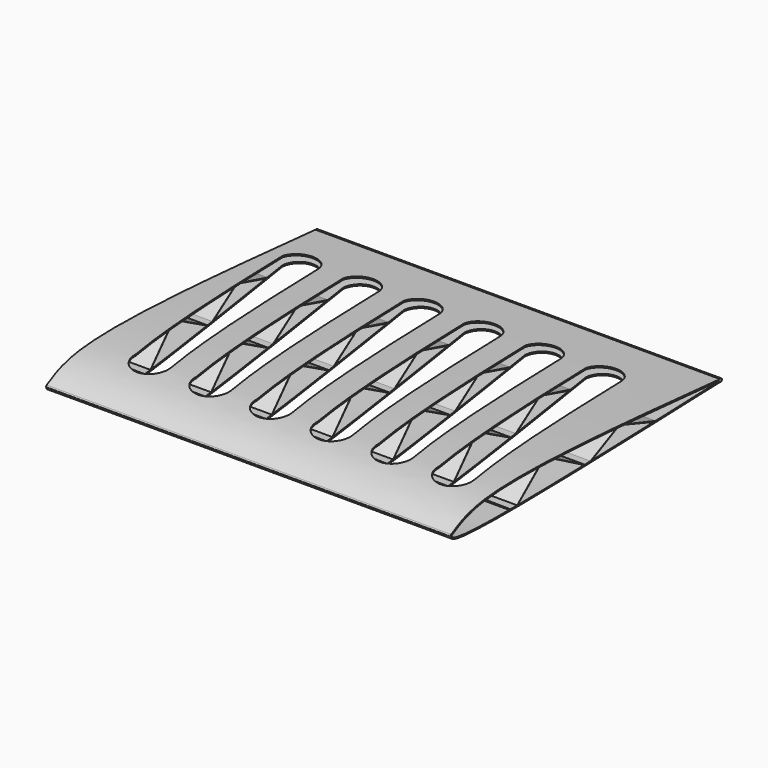
from build123d import *

# Parameters (mm, degrees)
F1_DEPTH      = 152.4
F3_DEPTH      = 152.4
F5_DEPTH      = 152.4
F7_DEPTH      = 152.4
F9_DEPTH      = 25.4
F9_DEPTH_BACK = 25.4


# Not quite as in the source:
# - the dataset's text gives a spline's control points without its knots; the knots are read off the source's solid


with BuildPart() as f1:
    # F0 (on Right) → F1 (new body)
    with BuildSketch(Plane.YZ):
        with BuildLine():
            add(Edge.make_bspline(
                [(-58.9602898603, 0.4442433921), (-58.1319828617, 0.9036602631), (-56.4650522891, 1.8284562183), (-53.665933112, 3.157433434), (-50.8685748203, 4.1483454801), (-48.2220596454, 4.8332931255), (-46.0009605563, 5.2847071379), (-43.505845475, 5.6643134941), (-39.7970976021, 6.0691924118), (-34.4832497676, 6.3982682422), (-27.1123389241, 6.536667424), (-16.089447743, 6.4144832315), (-0.3155135716, 5.7510734828), (21.0106659968, 4.3427449967), (43.935370548, 2.5263779626), (59.7506661768, 1.1795441585), (67.657842002, 0.5061678875)],
                knots=[0, 0, 0, 0, 0.0625, 0.125, 0.1875, 0.21875, 0.25, 0.28125, 0.3125, 0.375, 0.4375, 0.5, 0.625, 0.75, 0.875, 1, 1, 1, 1], degree=3))
            ThreePointArc((-58.9602898603, 0.4442433921), (-59.1623230661, 0.1771268563), (-59.1973622141, -0.1559510896))
            add(Edge.make_bspline(
                [(-59.1973622141, -0.1559510896), (-59.1586382603, -0.2760007197), (-59.0898574155, -0.4981328461), (-58.8919099657, -0.8348582239), (-58.6036542053, -1.1627799541), (-58.0769217377, -1.5065685431), (-57.1431398583, -1.8186205066), (-55.881573419, -2.082764659), (-53.7495870802, -2.3845446227), (-50.2565207316, -2.6781217899), (-44.8228964548, -2.9115194094), (-38.246663417, -3.0365419943), (-30.6295482411, -3.0633240776), (-19.223269712, -2.9812273008), (-2.8807115104, -2.682349235), (19.2331579069, -2.0882507198), (43.0156220319, -1.3372058258), (59.4265508418, -0.7842059692), (67.6318450558, -0.5077118308)],
                knots=[0, 0, 0, 0, 0.03125, 0.046875, 0.0625, 0.09375, 0.125, 0.15625, 0.1875, 0.25, 0.3125, 0.375, 0.4375, 0.5, 0.625, 0.75, 0.875, 1, 1, 1, 1], degree=3))
            ThreePointArc((67.6318450558, -0.5077118308), (68.5924443241, -0.0250694562), (67.657842002, 0.5061678875))
        make_face()
        with BuildLine():
            add(Edge.make_bspline(
                [(-58.7138921967, 0), (-58.5946909727, -0.3695403346), (-57.3555243321, -4.211127463), (8.2868285997, -1.9991749717), (67.6147366693, 0)],
                knots=[0, 0, 0, 0, 0.0961946865, 1, 1, 1, 1], degree=3))
            add(Edge.make_bspline(
                [(-58.7138921967, 0), (-55.1520692408, 1.9755495974), (-41.8991573794, 9.3262195537), (21.3582490553, 3.9392093748), (67.6147366693, 0)],
                knots=[0, 0, 0, 0, 0.2687577614, 1, 1, 1, 1], degree=3))
        make_face(mode=Mode.SUBTRACT)
    extrude(amount=F1_DEPTH)

    # F2 (on face) → F3 (join)
    with BuildSketch(Plane.YZ.offset(152.4)):
        Polygon((-42.8784973919, 5.4692113772), (-43.306030333, 5.4207709618), (-31.5003991127, -2.6227347553), (-30.8970212936, -2.6227347553), align=None)
    extrude(amount=-F3_DEPTH)

    # F4 (on face) → F5 (join)
    with BuildSketch(Plane.YZ.offset(152.4)):
        Polygon((-9.9641242996, 5.6611048058), (-10.1517588183, 5.6307056739), (3.7047350392, -1.9914695843), (4.0050991811, -1.9914695843), align=None)
        Polygon((-17.7478846163, 5.9763984755), (-27.9064550996, -2.5899412576), (-27.7177579701, -2.5948002003), (-17.4335390329, 5.9763984755), align=None)
    extrude(amount=-F5_DEPTH)

    # F6 (on face) → F7 (join)
    with BuildSketch(Plane.YZ.offset(152.4)):
        Polygon((19.0880838782, 4.061086569), (6.3000828959, -2.0995393861), (6.793865934, -2.1370307077), (19.4374024868, 4.061086569), align=None)
        Polygon((22.5569494069, 3.8362378255), (22.1231468022, 3.8362378255), (36.9006283581, -1.1861959938), (37.2741437614, -1.0062547589), align=None)
    extrude(amount=-F7_DEPTH)

    # F8 (on Top) → F9 (cut, two sides)
    with BuildSketch(Plane.XY) as f9_sk:
        with BuildLine():
            ThreePointArc((18.4947973731, 45.7572117448), (11.7873986866, 51.6837375641), (5.08, 45.7572117448))
            Line((5.08, 45.7572117448), (15.24, -36.119312048))
            ThreePointArc((15.24, -36.119312048), (21.9473986866, -43.7104705971), (28.6547973731, -36.119312048))
            Line((28.6547973731, -36.119312048), (18.4947973731, 45.7572117448))
        make_face()
        with BuildLine():
            Line((51.5147973731, -36.119312048), (41.3547973731, 45.7572117448))
            ThreePointArc((41.3547973731, 45.7572117448), (34.6473986866, 51.6837375641), (27.94, 45.7572117448))
            Line((27.94, 45.7572117448), (38.1, -36.119312048))
            ThreePointArc((38.1, -36.119312048), (44.8073986866, -43.7104705971), (51.5147973731, -36.119312048))
        make_face()
        with BuildLine():
            Line((74.3747973731, -36.119312048), (64.2147973731, 45.7572117448))
            ThreePointArc((64.2147973731, 45.7572117448), (57.5073986866, 51.6837375641), (50.8, 45.7572117448))
            Line((50.8, 45.7572117448), (60.96, -36.119312048))
            ThreePointArc((60.96, -36.119312048), (67.6673986866, -43.7104705971), (74.3747973731, -36.119312048))
        make_face()
        with BuildLine():
            Line((97.2347973731, -36.119312048), (87.0747973731, 45.7572117448))
            ThreePointArc((87.0747973731, 45.7572117448), (80.3673986866, 51.6837375641), (73.66, 45.7572117448))
            Line((73.66, 45.7572117448), (83.82, -36.119312048))
            ThreePointArc((83.82, -36.119312048), (90.5273986866, -43.7104705971), (97.2347973731, -36.119312048))
        make_face()
        with BuildLine():
            Line((120.0947973731, -36.119312048), (109.9347973731, 45.7572117448))
            ThreePointArc((109.9347973731, 45.7572117448), (103.2273986866, 51.6837375641), (96.52, 45.7572117448))
            Line((96.52, 45.7572117448), (106.68, -36.119312048))
            ThreePointArc((106.68, -36.119312048), (113.3873986866, -43.7104705971), (120.0947973731, -36.119312048))
        make_face()
        with BuildLine():
            Line((142.9547973731, -36.119312048), (132.7947973731, 45.7572117448))
            ThreePointArc((132.7947973731, 45.7572117448), (126.0873986866, 51.6837375641), (119.38, 45.7572117448))
            Line((119.38, 45.7572117448), (129.54, -36.119312048))
            ThreePointArc((129.54, -36.119312048), (136.2473986866, -43.7104705971), (142.9547973731, -36.119312048))
        make_face()
    extrude(amount=F9_DEPTH, mode=Mode.SUBTRACT)
    extrude(f9_sk.sketch, amount=-F9_DEPTH_BACK, mode=Mode.SUBTRACT)


solid = f1.part
